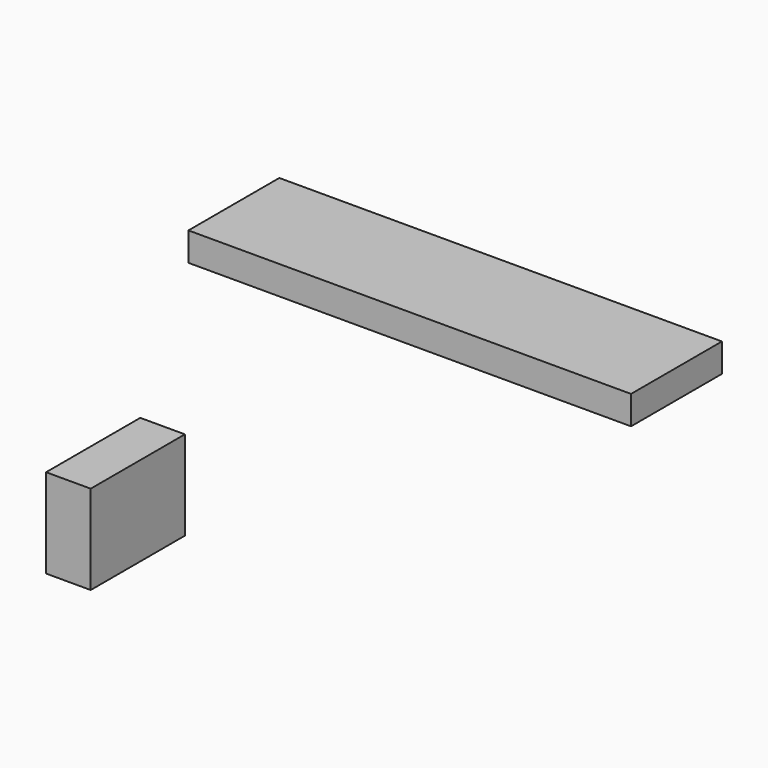
from build123d import *

# Parameters (mm, degrees)
F0_W     = 20.9442564005
F0_H     = 15.875
F1_DEPTH = 7.9375
F3_W     = 78.74
F3_H     = 20.2099310613
F4_DEPTH = 5.08


# Not quite as in the source:
# - the program builds the solid bodies; features that only make, move or delete a surface that nothing else refers to are left out


with BuildPart() as f1:
    # F0 (on Right) → F1 (new body)
    with BuildSketch(Plane.YZ):
        with Locations((-55.1829777162, -3.7632510066)):
            Rectangle(F0_W, F0_H)
    extrude(amount=F1_DEPTH)


with BuildPart() as f4:
    # F3 (on Top) → F4 (new body)
    with BuildSketch(Plane.XY):
        with Locations((10.4557741433, 12.2460403945)):
            Rectangle(F3_W, F3_H)
    extrude(amount=F4_DEPTH)


solid = Compound([f1.part, f4.part])
